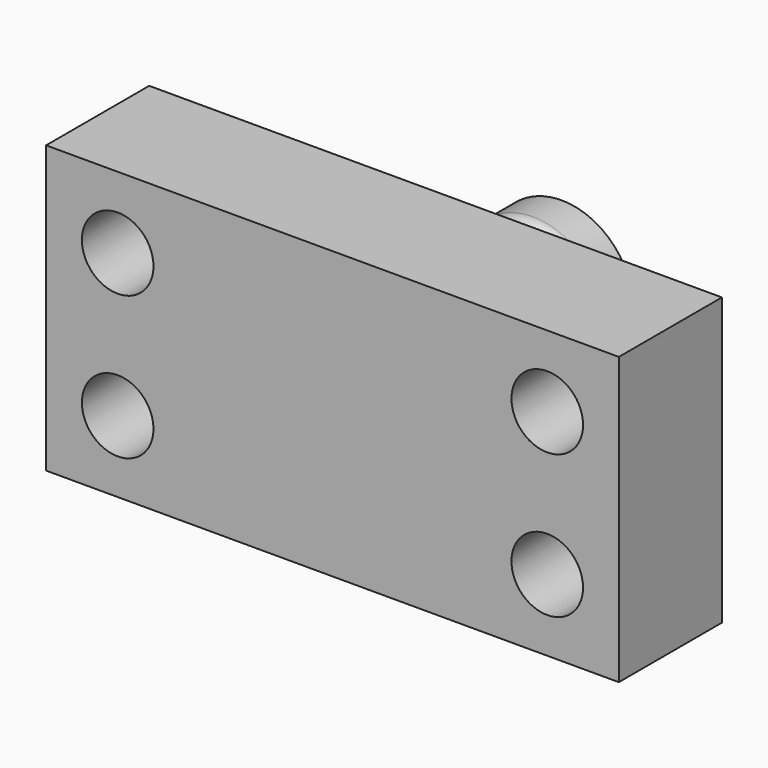
from build123d import *

# Parameters (mm, degrees)
F0_W     = 101.6
F0_H     = 50.8
F1_DEPTH = 25.4
F2_R     = 6.35
F3_DEPTH = 25.401
F4_W     = 12.7
F4_H     = 25.4
F6_W     = 8.9851264438
F6_H     = 6.35
F8_R     = 2.53999
F9_SIZE  = 2.54


# Not quite as in the source:
# - a fillet or chamfer is up to 0.001 mm smaller than in the source, because OpenCascade refuses the exact size


with BuildPart() as f1:
    # F0 (on Front) → F1 (new body)
    with BuildSketch(Plane.XZ):
        Rectangle(F0_W, F0_H)
    extrude(amount=F1_DEPTH)

    # F2 (on Front) → F3 (cut, through all)
    with BuildSketch(Plane.XZ):
        with Locations((-38.1, 12.7)):
            Circle(F2_R)
        with Locations((-38.1, -12.7)):
            Circle(F2_R)
        with Locations((38.1, -12.7)):
            Circle(F2_R)
        with Locations((38.1, 12.7)):
            Circle(F2_R)
    extrude(amount=F3_DEPTH, mode=Mode.SUBTRACT)

    # F4 (on Top) → F5 (revolve)
    with BuildSketch(Plane.XY):
        with Locations((6.35, 12.7)):
            Rectangle(F4_W, F4_H)
    revolve(axis=Axis((0, 12.7, 0), (0, 1, 0)))

    # F6 (on Top) → F7 (revolve, cut)
    with BuildSketch(Plane.XY):
        with Locations((-14.6525632219, 13.335)):
            Rectangle(F6_W, F6_H)
    revolve(axis=Axis((0, 6.6735967994, 0), (0, -1, 0)), mode=Mode.SUBTRACT)

    # F8 (radius 2.54 in the source; OpenCascade refuses exactly that, so slightly less here)
    f8_edges = [f1.edges().sort_by_distance(p)[0] for p in [
        (-12.7, 0, 0),
        (10.16, 10.16, 0),
        (-12.7, 16.51, 0),
    ]]
    fillet(f8_edges, radius=F8_R)

    # F9
    f9_edges = [f1.edges().sort_by_distance(p)[0] for p in [
        (0, 0, 25.4),
        (50.8, 0, 0),
        (0, 0, -25.4),
        (-50.8, 0, 0),
    ]]
    chamfer(f9_edges, length=F9_SIZE)


solid = f1.part
